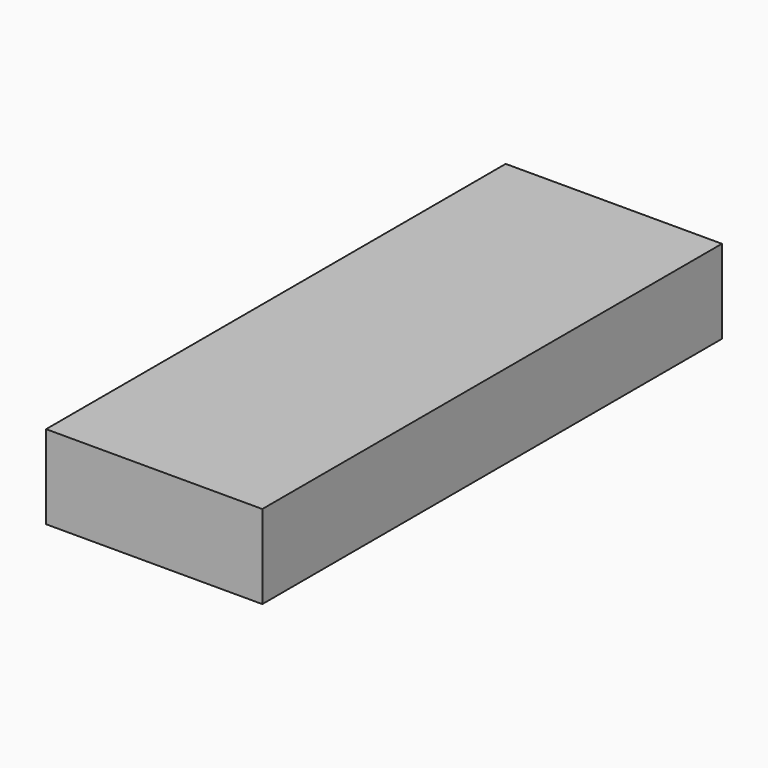
from build123d import *

# Parameters (mm, degrees)
F0_W     = 9.5608628471
F0_H     = 3.7018029252
F1_DEPTH = 25.4


# Not quite as in the source:
# - the program builds the solid bodies; features that only make, move or delete a surface that nothing else refers to are left out


with BuildPart() as f1:
    # F0 (on Front) → F1 (new body)
    with BuildSketch(Plane.XZ):
        with Locations((4.7804314236, 1.8509014626)):
            Rectangle(F0_W, F0_H)
    extrude(amount=F1_DEPTH)


solid = f1.part
